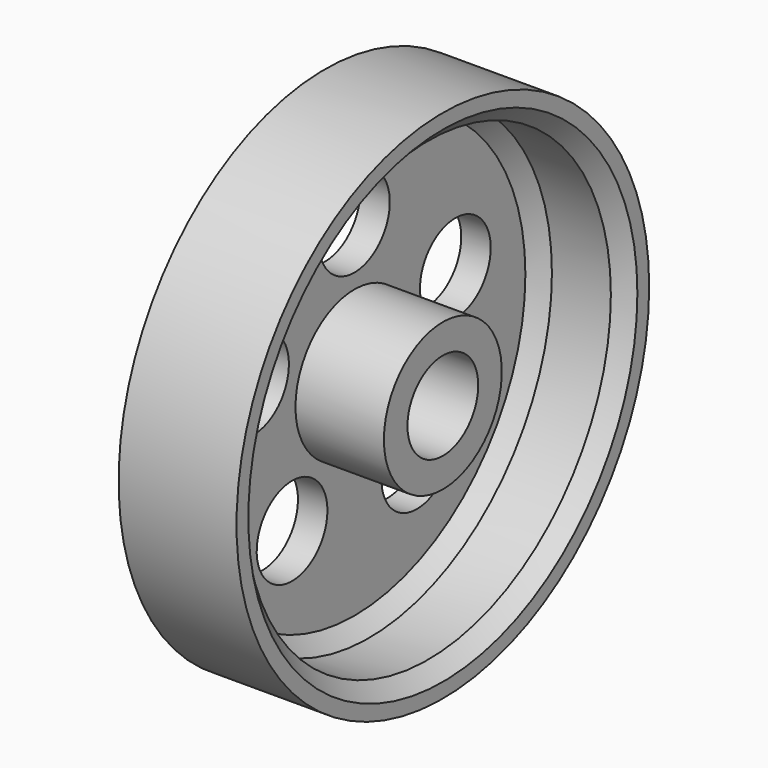
from build123d import *

# Parameters (mm, degrees)
F0_W            = 8
F0_H            = 17.5
F3_D            = 6
F4_T            = -2
F5_SIZE         = 1
F7_D            = 6
F7_COPIES_COUNT = 5


# Not quite as in the source:
# - a pattern or mirror of a feature is missing from the dataset's text; its kind, count and spacing are read off the source's solid


with BuildPart() as f1:
    # F0 (on Top) → F1 (revolve)
    with BuildSketch(Plane.XY):
        with Locations((4, 8.75)):
            Rectangle(F0_W, F0_H)
    revolve(axis=Axis((4, 0, 0), (1, 0, 0)))

    # F3 (through all)
    with Locations(Plane(origin=(0, 0, 0), x_dir=(0, 1, 0), z_dir=(-1, 0, 0))):
        with Locations((0, 0)):
            Hole(F3_D / 2)

    # F4
    f4_openings = [f1.faces().sort_by_distance(p)[0] for p in [
        (8, -17.005025, 0),
    ]]
    offset(amount=F4_T, openings=f4_openings)

    # F5
    f5_edges = [f1.edges().sort_by_distance(p)[0] for p in [
        (8, -15.5, 0),
        (5, 15.5, 0),
        (2, -15.5, 0),
    ]]
    chamfer(f5_edges, length=F5_SIZE)

    # F7 (through all)
    with Locations(Plane(origin=(0, 0, 0), x_dir=(0, 1, 0), z_dir=(-1, 0, 0))):
        with Locations((0, -9)):
            f7 = Hole(F7_D / 2)

    # F7_copies: F7 ×5 about axis
    f7_copies_axis = Axis((0, 0, 0), (1, 0, 0))
    for i in range(1, F7_COPIES_COUNT):
        add(f7.rotate(f7_copies_axis, i * 360 / F7_COPIES_COUNT), mode=Mode.SUBTRACT)


solid = f1.part
